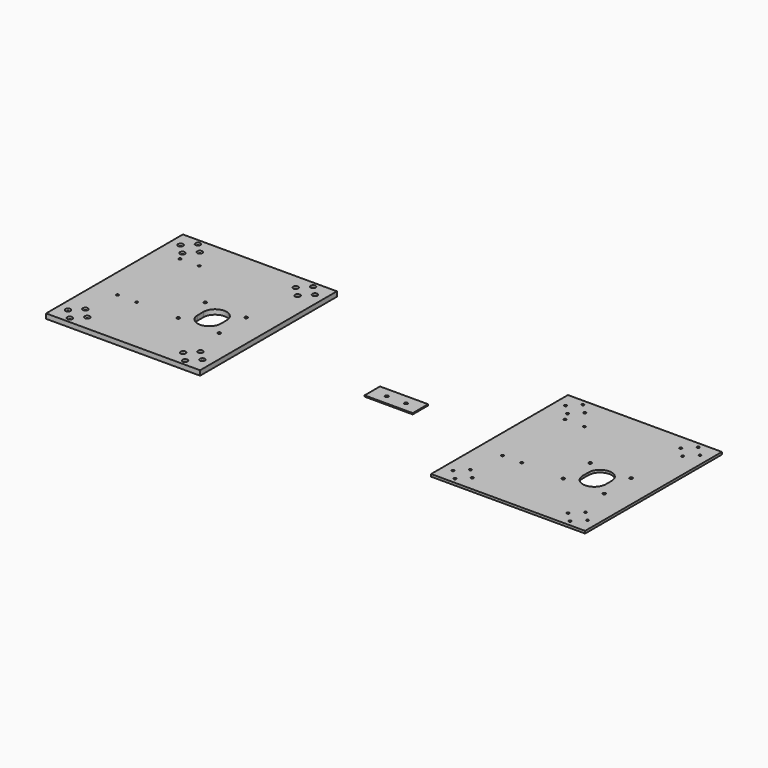
from build123d import *

# Parameters (mm, degrees)
F0_W           = 406.4
F0_H           = 451.4
F1_DEPTH       = 6.35
F2_D           = 6.6
F2_DEPTH       = 12
F2_CSINK_D     = 13.44
F2_CSINK_ANGLE = 90
F2_TIP         = 1.9828400428
F4_DEPTH       = 25.4
F5_D           = 6.5278
F5_DEPTH       = 20.1083333333
F5_TIP         = 1.9611489744
F6_W           = 406.4
F6_H           = 451.4
F7_DEPTH       = 12.7
F8_D           = 6.6
F8_DEPTH       = 18.8722
F8_CSINK_D     = 13.44
F8_CSINK_ANGLE = 90
F8_TIP         = 1.9828400428
F9_D           = 6.5278
F9_DEPTH       = 20.1083333333
F9_TIP         = 1.9611489744
F10_D          = 7.9375
F10_DEPTH      = 20.6459666667
F10_TIP        = 2.3846655818
F11_D          = 7.9375
F11_DEPTH      = 20.6459666667
F11_TIP        = 2.3846655818
F12_W          = 127
F12_H          = 50.8
F13_DEPTH      = 3.175
F14_D          = 8.4328
F14_DEPTH      = 20.6502
F14_TIP        = 2.5334687141


# Not quite as in the source:
# - a feature names something its author has since deleted; it is built from what else it names


with BuildPart() as f1:
    # F0 (on Top) → F1 (new body)
    with BuildSketch(Plane.XY):
        with Locations((203.2, 225.7)):
            Rectangle(F0_W, F0_H)
    extrude(amount=F1_DEPTH)

    # F2
    with Locations(Plane(origin=(0, 0, 0), x_dir=(1, 0, 0), z_dir=(0, 0, -1))):
        with Locations((355.12, -385.9), (329.62, -411.4), (355.12, -436.9), (380.62, -411.4), (76.78, -411.4), (51.28, -385.9), (25.78, -411.4), (51.28, -436.9), (51.28, -65.5), (25.78, -40), (51.28, -14.5), (76.78, -40), (329.62, -40), (355.12, -65.5), (380.62, -40), (355.12, -14.5)):
            CounterSinkHole(F2_D / 2, F2_CSINK_D / 2, depth=F2_DEPTH, counter_sink_angle=F2_CSINK_ANGLE)
            with Locations((0, 0, -(F2_DEPTH + F2_TIP / 2))):  # 118° drill point
                Cone(0, F2_D / 2, F2_TIP, mode=Mode.SUBTRACT)

    # F3 (on face) → F4 (cut)
    with BuildSketch(Plane.XY):
        with BuildLine():
            Line((248.92, 208.2331), (248.92, 189.1831))
            ThreePointArc((248.92, 189.1831), (279.4, 158.7031), (309.88, 189.1831))
            Line((309.88, 189.1831), (309.88, 208.2331))
            ThreePointArc((309.88, 208.2331), (279.4, 238.7131), (248.92, 208.2331))
        make_face()
    extrude(amount=F4_DEPTH, mode=Mode.SUBTRACT)

    # F5
    with Locations(Plane(origin=(0, 0, 0), x_dir=(1, 0, 0), z_dir=(0, 0, -1))):
        with Locations((63.5, -362.5), (114.3, -362.5), (63.5, -156.125), (114.3, -156.125)):
            Hole(F5_D / 2, depth=F5_DEPTH)
            with Locations((0, 0, -(F5_DEPTH + F5_TIP / 2))):  # 118° drill point
                Cone(0, F5_D / 2, F5_TIP, mode=Mode.SUBTRACT)

    # F11
    with Locations(Plane(origin=(0, 0, 0), x_dir=(1, 0, 0), z_dir=(0, 0, -1))):
        with Locations((333.375, -154.2581), (333.375, -243.1581), (225.425, -243.1581), (225.425, -154.2581)):
            Hole(F11_D / 2, depth=F11_DEPTH)
            with Locations((0, 0, -(F11_DEPTH + F11_TIP / 2))):  # 118° drill point
                Cone(0, F11_D / 2, F11_TIP, mode=Mode.SUBTRACT)


with BuildPart() as f7:
    # F6 (on Top) → F7 (new body)
    with BuildSketch(Plane.XY):
        with Locations((-871.8256354332, 299.2146255845)):
            Rectangle(F6_W, F6_H)
        with BuildLine():
            ThreePointArc((-765.145677681, 262.6977255845), (-795.625677681, 232.2177255845), (-826.105677681, 262.6977255845))
            Line((-826.105677681, 262.6977255845), (-826.105677681, 281.7477255845))
            ThreePointArc((-826.105677681, 281.7477255845), (-795.625677681, 312.2277255845), (-765.145677681, 281.7477255845))
            Line((-765.145677681, 281.7477255845), (-765.145677681, 262.6977255845))
        make_face(mode=Mode.SUBTRACT)
    extrude(amount=-F7_DEPTH)

    # F8
    with Locations(Plane.XY):
        with Locations((-1023.7456354332, 88.0146255845), (-1049.2456354332, 113.5146255845), (-998.2456354332, 113.5146255845), (-1023.7456354332, 139.0146255845), (-1023.7456354332, 459.4146255845), (-1049.2456354332, 484.9146255845), (-1023.7456354332, 510.4146255845), (-998.2456354332, 484.9146255845), (-719.9056354332, 459.4146255845), (-745.4056354332, 484.9146255845), (-694.4056354332, 484.9146255845), (-719.9056354332, 510.4146255845), (-719.9056354332, 139.0146255845), (-719.9056354332, 88.0146255845), (-694.4056354332, 113.5146255845), (-745.4056354332, 113.5146255845)):
            CounterSinkHole(F8_D / 2, F8_CSINK_D / 2, depth=F8_DEPTH, counter_sink_angle=F8_CSINK_ANGLE)
            with Locations((0, 0, -(F8_DEPTH + F8_TIP / 2))):  # 118° drill point
                Cone(0, F8_D / 2, F8_TIP, mode=Mode.SUBTRACT)

    # F9
    with Locations(Plane.XY):
        with Locations((-960.725677681, 229.6396255845), (-1011.525677681, 229.6396255845), (-960.725677681, 436.0146255845), (-1011.525677681, 436.0146255845)):
            Hole(F9_D / 2, depth=F9_DEPTH)
            with Locations((0, 0, -(F9_DEPTH + F9_TIP / 2))):  # 118° drill point
                Cone(0, F9_D / 2, F9_TIP, mode=Mode.SUBTRACT)

    # F10
    with Locations(Plane.XY):
        with Locations((-741.650677681, 227.7727255845), (-849.600677681, 227.7727255845), (-849.600677681, 316.6727255845), (-741.650677681, 316.6727255845)):
            Hole(F10_D / 2, depth=F10_DEPTH)
            with Locations((0, 0, -(F10_DEPTH + F10_TIP / 2))):  # 118° drill point
                Cone(0, F10_D / 2, F10_TIP, mode=Mode.SUBTRACT)


with BuildPart() as f13:
    # F12 (on Top) → F13 (new body)
    with BuildSketch(Plane.XY):
        with Locations((-266.7, 218.6746299267)):
            Rectangle(F12_W, F12_H)
    extrude(amount=F13_DEPTH)

    # F14
    with Locations(Plane(origin=(0, 0, 0), x_dir=(1, 0, 0), z_dir=(0, 0, -1))):
        with Locations((-241.3, -218.6746299267), (-292.1, -218.6746299267)):
            Hole(F14_D / 2, depth=F14_DEPTH)
            with Locations((0, 0, -(F14_DEPTH + F14_TIP / 2))):  # 118° drill point
                Cone(0, F14_D / 2, F14_TIP, mode=Mode.SUBTRACT)


with BuildPart() as f15_1:
    # F15: copy of F1
    add(f1.part)


solid = Compound([f1.part, f7.part, f13.part, f15_1.part])
